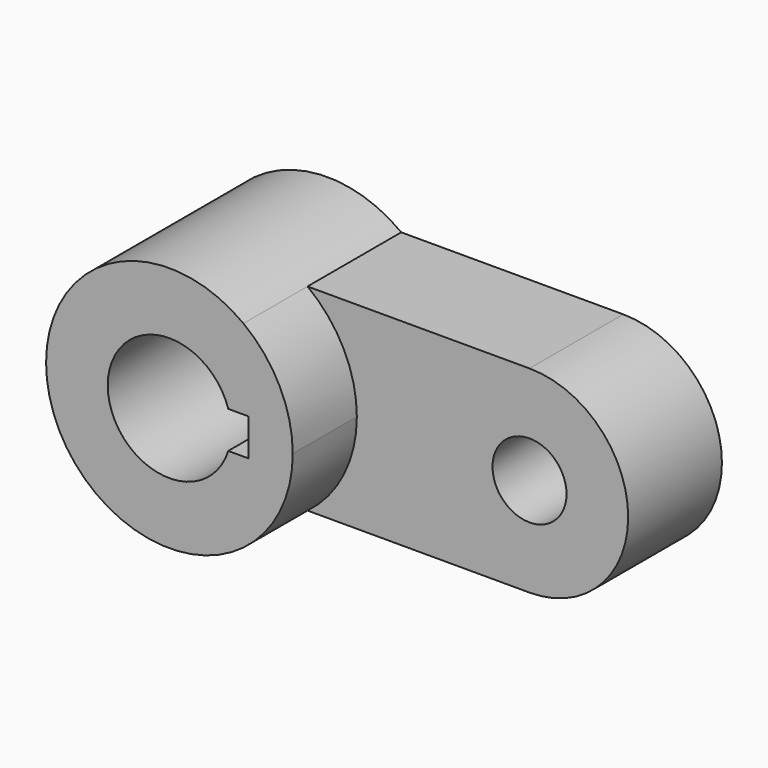
from build123d import *

# Parameters (mm, degrees)
F0_W     = 76.2
F0_H     = 50.8
F1_DEPTH = 30.1625
F3_DEPTH = 30.1752
F4_DEPTH = 20.6248
F5_DEPTH = 20.6248
F7_DEPTH = 50.8
F8_R     = 9.525
F9_DEPTH = 30.1752


with BuildPart() as f1:
    # F0 (on Front) → F1 (new body)
    with BuildSketch(Plane.XZ):
        with Locations((-38.1, 25.4)):
            Rectangle(F0_W, F0_H)
        with BuildLine():
            Line((0, 50.8), (0, 0))
            ThreePointArc((0, 0), (25.4, 25.4), (0, 50.8))
        make_face()
    extrude(amount=F1_DEPTH)

    # F2 (on face) → F3 (join)
    with BuildSketch(Plane.XZ.offset(30.1625)):
        with BuildLine():
            Line((-76.2, 50.8), (-57.15, 50.8))
            ThreePointArc((-57.15, 50.8), (-107.95, 25.4), (-57.15, 0))
            Line((-57.15, 0), (-76.2, 0))
            Line((-76.2, 0), (-76.2, 50.8))
        make_face()
    extrude(amount=-F3_DEPTH)

    # F2 (on face) → F4 (join)
    with BuildSketch(Plane.XZ.offset(30.1625)):
        with BuildLine():
            Line((-76.2, 50.8), (-57.15, 50.8))
            ThreePointArc((-57.15, 50.8), (-107.95, 25.4), (-57.15, 0))
            Line((-57.15, 0), (-76.2, 0))
            Line((-76.2, 0), (-76.2, 50.8))
        make_face()
    extrude(amount=F4_DEPTH)

    # F2 (on face) → F5 (join)
    with BuildSketch(Plane.XZ.offset(30.1625)):
        with BuildLine():
            ThreePointArc((-57.15, 0), (-47.8019366858, 11.2009683429), (-44.45, 25.4))
            ThreePointArc((-44.45, 25.4), (-47.8019366858, 39.5990316571), (-57.15, 50.8))
            Line((-57.15, 50.8), (-76.2, 50.8))
            Line((-76.2, 50.8), (-76.2, 0))
            Line((-76.2, 0), (-57.15, 0))
        make_face()
        with BuildLine():
            Line((-76.2, 50.8), (-57.15, 50.8))
            ThreePointArc((-57.15, 50.8), (-107.95, 25.4), (-57.15, 0))
            Line((-57.15, 0), (-76.2, 0))
            Line((-76.2, 0), (-76.2, 50.8))
        make_face()
    extrude(amount=F5_DEPTH)

    # F6 (on face) → F7 (cut)
    with BuildSketch(Plane.XZ.offset(50.7873)):
        with BuildLine():
            Line((-76.2, 25.4), (-60.325, 25.4))
            ThreePointArc((-60.325, 25.4), (-60.5088686027, 27.8091534761), (-61.0562151775, 30.1625))
            ThreePointArc((-61.0562151775, 30.1625), (-66.8082233443, 38.1988341754), (-76.2, 41.275))
            Line((-76.2, 41.275), (-76.2, 25.4))
        make_face()
        with BuildLine():
            Line((-55.7891130447, 25.4), (-60.325, 25.4))
            ThreePointArc((-60.325, 25.4), (-60.5088686027, 22.9908465239), (-61.0562151775, 20.6375))
            Line((-61.0562151775, 20.6375), (-55.7891130447, 20.6375))
            Line((-55.7891130447, 20.6375), (-55.7891130447, 25.4))
        make_face()
        with BuildLine():
            ThreePointArc((-61.0562151775, 20.6375), (-60.5088686027, 22.9908465239), (-60.325, 25.4))
            Line((-60.325, 25.4), (-76.2, 25.4))
            Line((-76.2, 25.4), (-76.2, 9.525))
            ThreePointArc((-76.2, 9.525), (-66.8082233443, 12.6011658246), (-61.0562151775, 20.6375))
        make_face()
        with BuildLine():
            ThreePointArc((-61.0562151775, 30.1625), (-60.5088686027, 27.8091534761), (-60.325, 25.4))
            Line((-60.325, 25.4), (-55.7891130447, 25.4))
            Line((-55.7891130447, 25.4), (-55.7891130447, 30.1625))
            Line((-55.7891130447, 30.1625), (-61.0562151775, 30.1625))
        make_face()
        with BuildLine():
            Line((-76.2, 9.525), (-76.2, 25.4))
            Line((-76.2, 25.4), (-76.2, 41.275))
            ThreePointArc((-76.2, 41.275), (-92.075, 25.4), (-76.2, 9.525))
        make_face()
    extrude(amount=-F7_DEPTH, mode=Mode.SUBTRACT)

    # F8 (on face) → F9 (cut)
    with BuildSketch(Plane.XZ.offset(30.1625)):
        with Locations((0, 25.4230257124)):
            Circle(F8_R)
    extrude(amount=-F9_DEPTH, mode=Mode.SUBTRACT)


solid = f1.part
